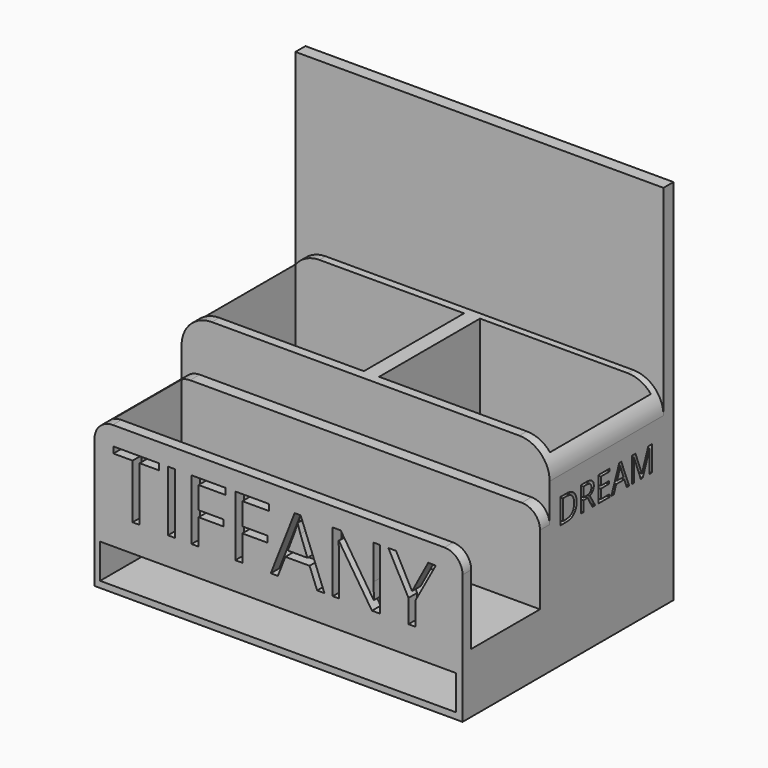
from build123d import *

# Parameters (mm, degrees)
F0_W          = 146.5508118272
F0_H          = 146.5508043766
F1_DEPTH      = 5
F2_W          = 146.5508118272
F2_H          = 18.8067741692
F3_DEPTH      = 100
F4_W          = 141.7780816555
F4_H          = 13.7566812336
F5_DEPTH      = 80
F6_W          = 72.9946568608
F6_H          = 56.6604238749
F6_W_2        = 73.5561549664
F7_DEPTH      = 60
F8_W          = 67.0427798759
F8_H          = 49.8609626666
F8_W_2        = 68.0534755811
F8_H_2        = 50.1978606917
F9_DEPTH      = 55
F10_W         = 146.5508118272
F10_H         = 43.3395761251
F11_DEPTH     = 40
F12_W         = 142.7303254604
F12_H         = 34.2267453671
F13_DEPTH     = 35
F14_R         = 5
F15_R         = 5
F16_T1_DEPTH  = 4.3165493011
F16_T3_DEPTH  = 4.7962814569
F16_T5_DEPTH  = 43.3395761251
F17_T1_DEPTH  = 86.8380934045
F18_TEXT_SIZE = 14.0083939562
F19_DEPTH     = 5
F20_TEXT_SIZE = 33.7624883833
F21_DEPTH     = 5


# Not quite as in the source:
# - a fillet or chamfer that OpenCascade refuses, or shapes differently, is made with other operations: its cross-section is extruded or revolved along the edge and cut away or added
# - a feature names something its author has since deleted; it is built from what else it names
# - Text() gives the source's letters only with a copy of the font that has no kerning and outlines rounded to 1/6400 em; it was checked with that copy


with BuildPart() as f1:
    # F0 (on Front) → F1 (new body)
    with BuildSketch(Plane.XZ):
        with Locations((0.2807490528, -0.4211217165)):
            Rectangle(F0_W, F0_H)
    extrude(amount=F1_DEPTH)

    # F2 (on face) → F3 (join)
    with BuildSketch(Plane.XZ.offset(5)):
        with Locations((0.2807490528, -64.2931368202)):
            Rectangle(F2_W, F2_H)
    extrude(amount=F3_DEPTH)

    # F4 (on face) → F5 (cut)
    with BuildSketch(Plane.XZ.offset(105)):
        with Locations((0.140376389, -64.2914455384)):
            Rectangle(F4_W, F4_H)
    extrude(amount=-F5_DEPTH, mode=Mode.SUBTRACT)

    # F6 (on face) → F7 (join)
    with BuildSketch(Plane.XY.offset(-54.8897497356)):
        with Locations((-36.4973284304, -33.3302119374)):
            Rectangle(F6_W, F6_H)
        with Locations((36.7780774832, -33.3302119374)):
            Rectangle(F6_W_2, F6_H)
    extrude(amount=F7_DEPTH)

    # F8 (on face) → F9 (cut)
    with BuildSketch(Plane.XY.offset(5.1102502644)):
        with Locations((-36.8903741473, -33.0240610056)):
            Rectangle(F8_W, F8_H)
        with Locations((36.7219266482, -32.855611993)):
            Rectangle(F8_W_2, F8_H_2)
    extrude(amount=-F9_DEPTH, mode=Mode.SUBTRACT)

    # F10 (on face) → F11 (join)
    with BuildSketch(Plane.XY.offset(-54.8897497356)):
        with Locations((0.2807490528, -83.3302119374)):
            Rectangle(F10_W, F10_H)
    extrude(amount=F11_DEPTH)

    # F12 (on face) → F13 (cut)
    with BuildSketch(Plane.XY.offset(-14.8897497356)):
        with Locations((2.1909922361, -83.5700780153)):
            Rectangle(F12_W, F12_H)
    extrude(amount=-F13_DEPTH, mode=Mode.SUBTRACT)

    # F14
    f14_edges = [f1.edges().sort_by_distance(p)[0] for p in [
        (-36.890374, -8.09358, -49.88975),
        (-70.411764, -33.024061, -49.88975),
        (-36.890374, -57.954542, -49.88975),
        (-3.368984, -33.024061, -49.88975),
    ]]
    fillet(f14_edges, radius=F14_R)

    # F15
    f15_edges = [f1.edges().sort_by_distance(p)[0] for p in [
        (36.721927, -7.756682, -49.88975),
        (2.695189, -32.855612, -49.88975),
        (36.721927, -57.954542, -49.88975),
        (70.748664, -32.855612, -49.88975),
    ]]
    fillet(f15_edges, radius=F15_R)

    # F16: fillet of radius 7.2426406871 on 3 edges, made by hand

    # F16_s2 → F16_t1 (cut)
    with BuildSketch(Plane.XZ.offset(100.6834506989)):
        with BuildLine():
            ThreePointArc((73.5561549664, -22.1323904227), (71.4348346228, -17.0110700792), (66.3135142792, -14.8897497356))
            Line((66.3135142792, -14.8897497356), (66.3135142792, -14.7448969219))
            Line((66.3135142792, -14.7448969219), (73.7010077801, -14.7448969219))
            Line((73.7010077801, -14.7448969219), (73.7010077801, -22.1323904227))
            Line((73.7010077801, -22.1323904227), (73.5561549664, -22.1323904227))
        make_face()
    extrude(amount=F16_T1_DEPTH, mode=Mode.SUBTRACT)

    # F16_s4 → F16_t3 (cut)
    with BuildSketch(Plane.XZ.offset(61.6604238749)):
        with BuildLine():
            ThreePointArc((73.5561549664, -22.1323904227), (71.4348346228, -17.0110700792), (66.3135142792, -14.8897497356))
            Line((66.3135142792, -14.8897497356), (66.3135142792, -14.7448969219))
            Line((66.3135142792, -14.7448969219), (73.7010077801, -14.7448969219))
            Line((73.7010077801, -14.7448969219), (73.7010077801, -22.1323904227))
            Line((73.7010077801, -22.1323904227), (73.5561549664, -22.1323904227))
        make_face()
    extrude(amount=F16_T3_DEPTH, mode=Mode.SUBTRACT)

    # F16_s6 → F16_t5 (cut)
    with BuildSketch(Plane.XZ.offset(61.6604238749)):
        with BuildLine():
            ThreePointArc((-72.9946568608, -22.1323904227), (-70.8733365173, -17.0110700792), (-65.7520161737, -14.8897497356))
            Line((-65.7520161737, -14.8897497356), (-65.7520161737, -14.7448969219))
            Line((-65.7520161737, -14.7448969219), (-73.1395096746, -14.7448969219))
            Line((-73.1395096746, -14.7448969219), (-73.1395096746, -22.1323904227))
            Line((-73.1395096746, -22.1323904227), (-72.9946568608, -22.1323904227))
        make_face()
    extrude(amount=F16_T5_DEPTH, mode=Mode.SUBTRACT)

    # F17: fillet of radius 12.0710678119 on 2 edges, made by hand

    # F17_s2 → F17_t1 (cut)
    with BuildSketch(Plane.XZ.offset(5)):
        with BuildLine():
            ThreePointArc((-60.923589049, 5.1102502644), (-69.4591229549, 1.5747163585), (-72.9946568608, -6.9608175475))
            Line((-72.9946568608, -6.9608175475), (-72.9946568608, 5.1102502644))
            Line((-72.9946568608, 5.1102502644), (-60.923589049, 5.1102502644))
        make_face()
        with BuildLine():
            ThreePointArc((61.4850871545, 5.1102502644), (70.0206210604, 1.5747163585), (73.5561549664, -6.9608175475))
            Line((73.5561549664, -6.9608175475), (73.5561549664, 5.1102502644))
            Line((73.5561549664, 5.1102502644), (61.4850871545, 5.1102502644))
        make_face()
    extrude(amount=F17_T1_DEPTH, mode=Mode.SUBTRACT)

    # F18 (on face) → F19 (cut)
    with BuildSketch(Plane.YZ.offset(73.5561549664)):
        with Locations((-57.6044102539, -24.6326476336)):
            Text('DREAM', F18_TEXT_SIZE, font='Open Sans', text_align=(TextAlign.LEFT, TextAlign.BOTTOM))
    extrude(amount=-F19_DEPTH, mode=Mode.SUBTRACT)

    # F20 (on face) → F21 (cut)
    with BuildSketch(Plane.XZ.offset(105)):
        with Locations((-65.7520161737, -46.4413820587)):
            Text('TIFFANY', F20_TEXT_SIZE, font='Open Sans', text_align=(TextAlign.LEFT, TextAlign.BOTTOM))
    extrude(amount=-F21_DEPTH, mode=Mode.SUBTRACT)


solid = f1.part
